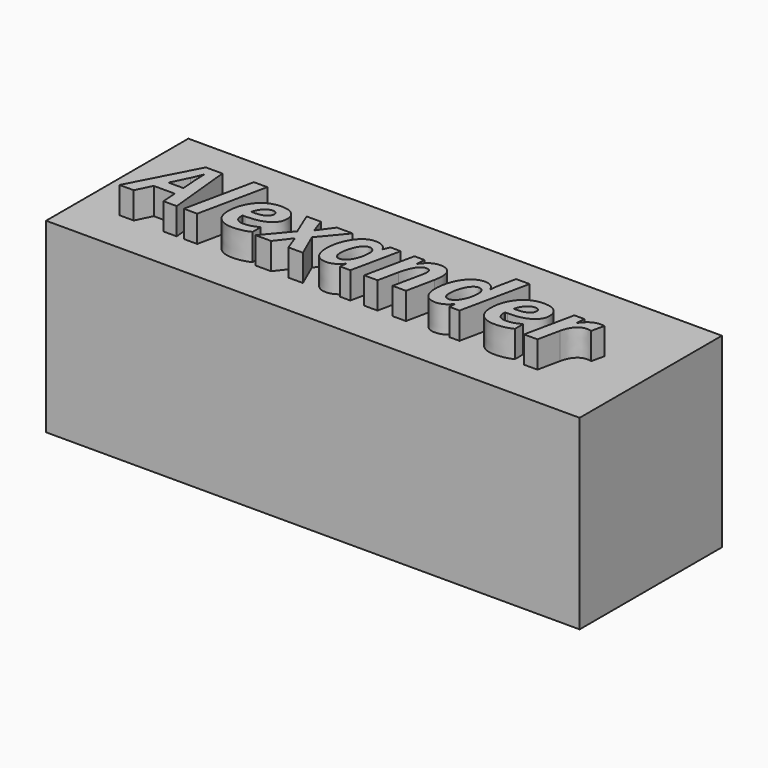
from build123d import *

# Parameters (mm, degrees)
F0_W         = 60
F0_H         = 20
F1_DEPTH     = 20.94763
F2_TEXT_SIZE = 10.2449175604
F3_DEPTH     = 3


# Not quite as in the source:
# - Text() gives the source's letters only with a copy of the font that has no kerning and outlines rounded to 1/6400 em; it was checked with that copy


with BuildPart() as f1:
    # F0 (on Top) → F1 (new body)
    with BuildSketch(Plane.XY):
        Rectangle(F0_W, F0_H)
    extrude(amount=F1_DEPTH)

    # F2 (on face) → F3 (join)
    with BuildSketch(Plane.XY.offset(20.94763)):
        with Locations((-25, -5.1631147653)):
            Text('Alexander', F2_TEXT_SIZE, font='Open Sans', font_style=FontStyle.BOLDITALIC, text_align=(TextAlign.LEFT, TextAlign.BOTTOM))
    extrude(amount=F3_DEPTH)


solid = f1.part
